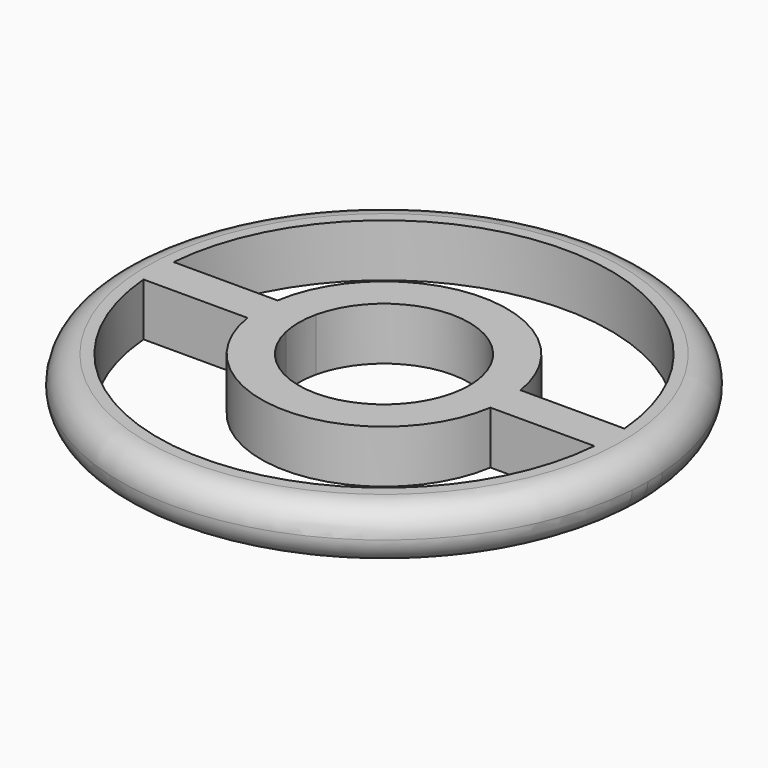
from build123d import *

# Parameters (mm, degrees)
F1_DEPTH = 7
F3_R     = 3.49999


# Not quite as in the source:
# - a fillet or chamfer that OpenCascade refuses, or shapes differently, is made with other operations: its cross-section is extruded or revolved along the edge and cut away or added
# - a fillet or chamfer is up to 0.001 mm smaller than in the source, because OpenCascade refuses the exact size


with BuildPart() as f1:
    # F0 (on Top) → F1 (new body)
    with BuildSketch(Plane.XY):
        with BuildLine():
            ThreePointArc((-29.8956518578, 2.5), (0, 30), (29.8956518578, 2.5))
            Line((29.8956518578, 2.5), (34.9106001094, 2.5))
            ThreePointArc((34.9106001094, 2.5), (0, 35), (-34.9106001094, 2.5))
            Line((-34.9106001094, 2.5), (-29.8956518578, 2.5))
        make_face()
        with BuildLine():
            Line((34.9106001094, 2.5), (29.8956518578, 2.5))
            ThreePointArc((29.8956518578, 2.5), (29.9739016123, 1.2510883797), (30, 0))
            ThreePointArc((30, 0), (29.9739016123, -1.2510883797), (29.8956518578, -2.5))
            Line((29.8956518578, -2.5), (34.9106001094, -2.5))
            ThreePointArc((34.9106001094, -2.5), (34.9776428868, -1.2507989787), (35, 0))
            ThreePointArc((35, 0), (34.9776428868, 1.2507989787), (34.9106001094, 2.5))
        make_face()
        with BuildLine():
            Line((34.9106001094, -2.5), (29.8956518578, -2.5))
            ThreePointArc((29.8956518578, -2.5), (0, -30), (-29.8956518578, -2.5))
            Line((-29.8956518578, -2.5), (-34.9106001094, -2.5))
            ThreePointArc((-34.9106001094, -2.5), (0, -35), (34.9106001094, -2.5))
        make_face()
        with BuildLine():
            ThreePointArc((-29.8956518578, -2.5), (-30, 0), (-29.8956518578, 2.5))
            Line((-29.8956518578, 2.5), (-34.9106001094, 2.5))
            ThreePointArc((-34.9106001094, 2.5), (-35, 0), (-34.9106001094, -2.5))
            Line((-34.9106001094, -2.5), (-29.8956518578, -2.5))
        make_face()
        with BuildLine():
            ThreePointArc((-16.1071412734, -2.5), (-16.3, 0), (-16.1071412734, 2.5))
            Line((-16.1071412734, 2.5), (-29.8956518578, 2.5))
            ThreePointArc((-29.8956518578, 2.5), (-30, 0), (-29.8956518578, -2.5))
            Line((-29.8956518578, -2.5), (-16.1071412734, -2.5))
        make_face()
        with BuildLine():
            ThreePointArc((-11.0199818512, -2.5), (-11.3, 0), (-11.0199818512, 2.5))
            Line((-11.0199818512, 2.5), (-16.1071412734, 2.5))
            ThreePointArc((-16.1071412734, 2.5), (-16.3, 0), (-16.1071412734, -2.5))
            Line((-16.1071412734, -2.5), (-11.0199818512, -2.5))
        make_face()
        with BuildLine():
            ThreePointArc((-11.0199818512, 2.5), (0, 11.3), (11.0199818512, 2.5))
            Line((11.0199818512, 2.5), (16.1071412734, 2.5))
            ThreePointArc((16.1071412734, 2.5), (0, 16.3), (-16.1071412734, 2.5))
            Line((-16.1071412734, 2.5), (-11.0199818512, 2.5))
        make_face()
        with BuildLine():
            Line((16.1071412734, -2.5), (11.0199818512, -2.5))
            ThreePointArc((11.0199818512, -2.5), (0, -11.3), (-11.0199818512, -2.5))
            Line((-11.0199818512, -2.5), (-16.1071412734, -2.5))
            ThreePointArc((-16.1071412734, -2.5), (0, -16.3), (16.1071412734, -2.5))
        make_face()
        with BuildLine():
            Line((29.8956518578, 2.5), (16.1071412734, 2.5))
            ThreePointArc((16.1071412734, 2.5), (16.2517137982, 1.2537139315), (16.3, 0))
            ThreePointArc((16.3, 0), (16.2517137982, -1.2537139315), (16.1071412734, -2.5))
            Line((16.1071412734, -2.5), (29.8956518578, -2.5))
            ThreePointArc((29.8956518578, -2.5), (29.9739016123, -1.2510883797), (30, 0))
            ThreePointArc((30, 0), (29.9739016123, 1.2510883797), (29.8956518578, 2.5))
        make_face()
        with BuildLine():
            ThreePointArc((11.0199818512, 2.5), (11.2297772667, 1.2578165768), (11.3, 0))
            ThreePointArc((11.3, 0), (11.2297772667, -1.2578165768), (11.0199818512, -2.5))
            Line((11.0199818512, -2.5), (16.1071412734, -2.5))
            ThreePointArc((16.1071412734, -2.5), (16.2517137982, -1.2537139315), (16.3, 0))
            ThreePointArc((16.3, 0), (16.2517137982, 1.2537139315), (16.1071412734, 2.5))
            Line((16.1071412734, 2.5), (11.0199818512, 2.5))
        make_face()
    extrude(amount=F1_DEPTH)

    # F2: fillet of radius 3.5 on 1 edges, made by hand

    # F2_s1 → F2_t2 (revolve, cut)
    with BuildSketch(Plane(origin=(0, 0, 0), x_dir=(0, 0, 1), z_dir=(0.0714285714, 0.9974457174, 0))):
        with BuildLine():
            ThreePointArc((3.5, -35), (5.9748737342, -33.9748737342), (7, -31.5))
            Line((7, -31.5), (7, -35))
            Line((7, -35), (3.5, -35))
        make_face()
    revolve(axis=Axis((0, 0, 7), (0, 0, 1)), mode=Mode.SUBTRACT)

    # F3 (radius 3.5 in the source; OpenCascade refuses exactly that, so slightly less here)
    f3_edges = [f1.edges().sort_by_distance(p)[0] for p in [
        (34.9106, -2.5, 0),
    ]]
    fillet(f3_edges, radius=F3_R)


solid = f1.part
